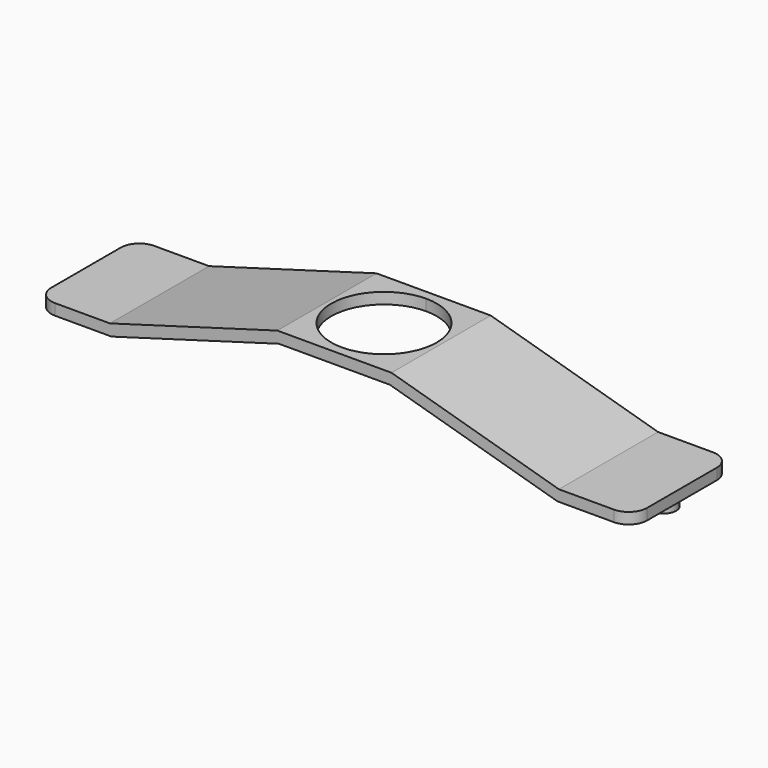
from build123d import *

# Parameters (mm, degrees)
F2_DEPTH = 16.75
F4_DEPTH = 16.001
F5_R     = 3.429
F6_R     = 3.429
F7_DEPTH = 3
F8_R     = 5
F9_R     = 5
F10_R    = 5
F11_R    = 5


with BuildPart() as f2:
    # F1 (on Front) → F2 (new body, symmetric)
    with BuildSketch(Plane.XZ):
        Polygon((-84.0640169114, 3), (-84.0640169114, 0), (-63.7959806109, 0), (-18.5640169114, 13), (11.4359830886, 13), (56.667946788, 0), (76.9359830886, 0), (76.9359830886, 3), (57.0905048336, 3), (11.8585411342, 16), (-18.986574957, 16), (-64.2185386565, 3), align=None)
    extrude(amount=F2_DEPTH, both=True)

    # F3 (on face) → F4 (cut, through all)
    with BuildSketch(Plane.XY.offset(16)):
        with BuildLine():
            ThreePointArc((-3.5640168758, -14.25), (6.5122547331, -10.0762716193), (10.6859830886, 0))
            ThreePointArc((10.6859830886, 0), (6.5122547205, 10.0762716319), (-3.5640169114, 14.25))
            ThreePointArc((-3.5640169114, 14.25), (-17.8140169114, -1.78e-08), (-3.5640168758, -14.25))
        make_face()
    extrude(amount=-F4_DEPTH, mode=Mode.SUBTRACT)

    # F5 (on face) + F6 (on face) → F7 (join)
    with BuildSketch(Plane(origin=(0, 0, 0), x_dir=(1, 0, 0), z_dir=(0, 0, -1))):
        with Locations((-79.0640169114, 0)):
            Circle(F5_R)
    with BuildSketch(Plane(origin=(0, 0, 0), x_dir=(1, 0, 0), z_dir=(0, 0, -1))):
        with Locations((71.9359830886, 0)):
            Circle(F6_R)
    extrude(amount=F7_DEPTH)

    # F8
    f8_edges = [f2.edges().sort_by_distance(p)[0] for p in [
        (-84.064017, -16.75, 1.5),
    ]]
    fillet(f8_edges, radius=F8_R)

    # F9
    f9_edges = [f2.edges().sort_by_distance(p)[0] for p in [
        (-84.064017, 16.75, 1.5),
    ]]
    fillet(f9_edges, radius=F9_R)

    # F10
    f10_edges = [f2.edges().sort_by_distance(p)[0] for p in [
        (76.935983, -16.75, 1.5),
    ]]
    fillet(f10_edges, radius=F10_R)

    # F11
    f11_edges = [f2.edges().sort_by_distance(p)[0] for p in [
        (76.935983, 16.75, 1.5),
    ]]
    fillet(f11_edges, radius=F11_R)


solid = f2.part
